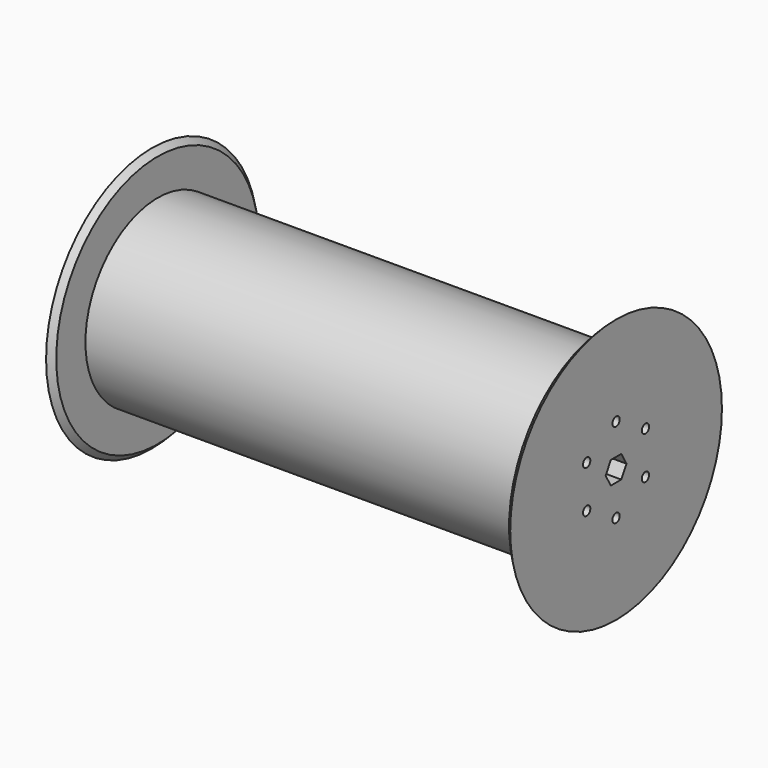
from build123d import *

# Parameters (mm, degrees)
F0_R          = 50.8
F1_DEPTH      = 254
F3_DEPTH      = 50.801
F4_R          = 44.45
F1_FACE1_R    = 50.8
F5_DEPTH      = 254.001
F6_R          = 5.08
F7_R          = 44.196
F8_DEPTH      = 0.127
F8_DEPTH_BACK = 9.525
F9_R          = 76.2
F10_DEPTH     = 3.175
F13_D         = 5.1054
F13_DEPTH     = 12.7
F13_TIP       = 1.5338169022


# Not quite as in the source:
# - a fillet or chamfer that OpenCascade refuses, or shapes differently, is made with other operations: its cross-section is extruded or revolved along the edge and cut away or added


with BuildPart() as f1:
    # F0 (on Right) → F1 (new body)
    with BuildSketch(Plane.YZ):
        Circle(F0_R)
    extrude(amount=F1_DEPTH)

    # F2 (on Front) → F3 (cut, through all)
    with BuildSketch(Plane.XZ):
        Polygon((38.1, 38.1), (25.4, 38.1), (25.4, 25.4), (25.4, 4.2028785683), (25.4, -38.1), (228.6, -38.1), (228.6, 12.7), (215.9, 12.7), (215.9, 38.1), (203.2, 38.1), (203.2, 12.7), (190.5, 12.7), (190.5, 38.1), (177.8, 38.1), (177.8, 12.7), (165.1, 12.7), (165.1, 38.1), (152.4, 38.1), (152.4, 12.7), (139.7, 12.7), (139.7, 38.1), (127, 38.1), (127, 12.7), (114.3, 12.7), (114.3, 38.1), (101.6, 38.1), (101.6, 12.7), (88.9, 12.7), (88.9, 38.1), (76.2, 38.1), (76.2, 12.7), (63.5, 12.7), (63.5, 38.1), (50.8, 38.1), (50.8, 12.7), (38.1, 12.7), align=None)
    extrude(amount=-F3_DEPTH, mode=Mode.SUBTRACT)

    # F4 (on face) + F1_face1 (on face) → F5 (cut, through all)
    with BuildSketch(Plane.YZ.offset(254)):
        Circle(F4_R)
    with BuildSketch(Plane(origin=(0, 0, 0), x_dir=(0, 1, 0), z_dir=(-1, 0, 0))):
        Circle(F1_FACE1_R)
    extrude(amount=-F5_DEPTH, dir=(1, 0, 0), mode=Mode.SUBTRACT)

    # F6
    f6_edges = [f1.edges().sort_by_distance(p)[0] for p in [
        (38.1, 45.891992, 12.7),
        (50.8, 45.891992, 12.7),
        (76.2, 45.891992, 12.7),
        (101.6, 45.891992, 12.7),
        (127, 45.891992, 12.7),
        (152.4, 45.891992, 12.7),
        (177.8, 45.891992, 12.7),
        (203.2, 45.891992, 12.7),
        (63.5, 45.891992, 12.7),
        (88.9, 45.891992, 12.7),
        (114.3, 45.891992, 12.7),
        (139.7, 45.891992, 12.7),
        (165.1, 45.891992, 12.7),
        (190.5, 45.891992, 12.7),
        (215.9, 45.891992, 12.7),
        (38.1, 28.248146, 38.1),
        (63.5, 28.248146, 38.1),
        (50.8, 28.248146, 38.1),
        (76.2, 28.248146, 38.1),
        (88.9, 28.248146, 38.1),
        (101.6, 28.248146, 38.1),
        (114.3, 28.248146, 38.1),
        (127, 28.248146, 38.1),
        (152.4, 28.248146, 38.1),
        (165.1, 28.248146, 38.1),
        (139.7, 28.248146, 38.1),
        (177.8, 28.248146, 38.1),
        (203.2, 28.248146, 38.1),
        (190.5, 28.248146, 38.1),
        (215.9, 28.248146, 38.1),
        (25.4, 28.248146, 38.1),
    ]]
    fillet(f6_edges, radius=F6_R)


with BuildPart() as f8:
    # F7 (on face) → F8 (new body, two sides)
    with BuildSketch(Plane.YZ.offset(254)) as f8_sk:
        Circle(F7_R)
        Polygon((7.3323484187, 0), (3.6661742094, -6.35), (-3.6661742094, -6.35), (-7.3323484187, 0), (-3.6661742094, 6.35), (3.6661742094, 6.35), align=None, mode=Mode.SUBTRACT)
    extrude(amount=F8_DEPTH)
    extrude(f8_sk.sketch, amount=-F8_DEPTH_BACK)

    # F9 (on face) → F10 (join)
    with BuildSketch(Plane.YZ.offset(254.127)):
        Circle(F9_R)
        Polygon((7.3323484187, 0), (3.6661742094, -6.35), (-3.6661742094, -6.35), (-7.3323484187, 0), (-3.6661742094, 6.35), (3.6661742094, 6.35), align=None, mode=Mode.SUBTRACT)
    extrude(amount=F10_DEPTH)

    # F12: chamfer of 5.08 on 1 edges, made by hand

    # F12_s1 → F12_t2 (revolve, cut)
    with BuildSketch(Plane.XY):
        Polygon((254.127, 71.12), (259.207, 76.2), (254.127, 76.2), align=None)
    revolve(axis=Axis((254.127, 0, 0), (1, 0, 0)), mode=Mode.SUBTRACT)

    # F13
    with Locations(Plane.YZ.offset(257.302)):
        with Locations((0, 23.8125), (20.6222299276, 11.90625), (20.6222299276, -11.90625), (0, -23.8125), (-20.6222299276, -11.90625), (-20.6222299276, 11.90625)):
            Hole(F13_D / 2, depth=F13_DEPTH)
            with Locations((0, 0, -(F13_DEPTH + F13_TIP / 2))):  # 118° drill point
                Cone(0, F13_D / 2, F13_TIP, mode=Mode.SUBTRACT)


with BuildPart() as f15_1:
    # F15: instance of F8
    add(f8.part.mirror(Plane(origin=(127, 0, 0), x_dir=(0, 1, 0), z_dir=(-1, 0, 0))))


solid = Compound([f1.part, f8.part, f15_1.part])
